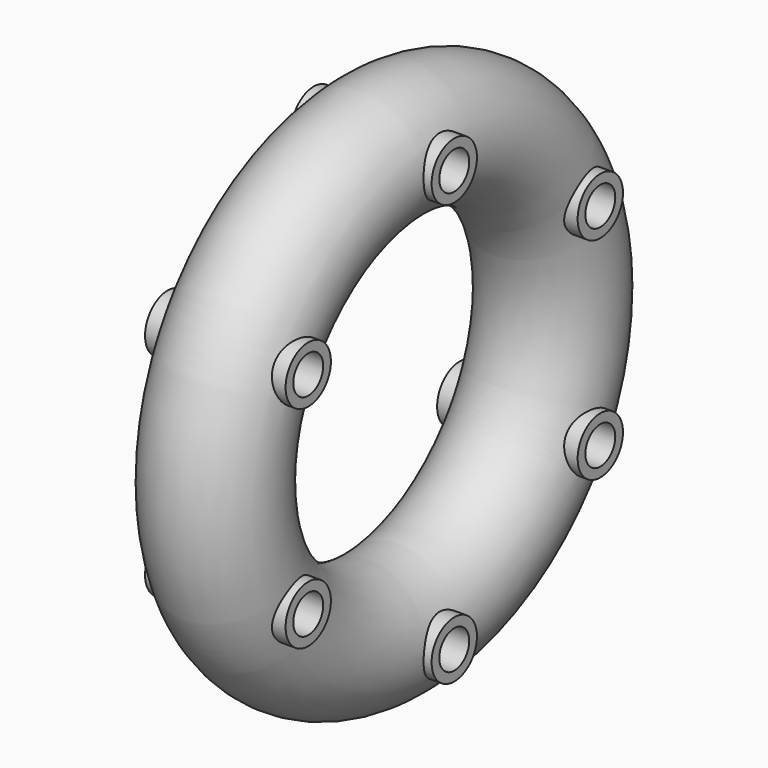
from build123d import *
from build123d import SkipClean  # not in build123d's __all__

# Parameters (mm, degrees)
F0_R          = 27.5
F2_R          = 12.5
F3_DEPTH      = 27.5010001
F3_DEPTH_BACK = 27.501
F4_R          = 12.5
F4_R_2        = 8.25
F5_DEPTH      = 31
F5_DEPTH_BACK = 31


with BuildPart() as f1:
    # F0 (on Front) → F1 (revolve)
    with BuildSketch(Plane.XZ):
        with Locations((0, 93)):
            Circle(F0_R)
    revolve(axis=Axis((3.4763067961, 0, 0), (1, 0, 0)))

    # F2 (on Right) → F3 (cut, two sides)
    with BuildSketch(Plane.YZ) as f3_sk:
        with Locations((0, 93)):
            Circle(F2_R)
        with Locations((-80.540362552, 46.5)):
            Circle(F2_R)
        with Locations((-80.540362552, -46.5)):
            Circle(F2_R)
        with Locations((0, -93)):
            Circle(F2_R)
        with Locations((80.540362552, -46.5)):
            Circle(F2_R)
        with Locations((80.540362552, 46.5)):
            Circle(F2_R)
    with SkipClean():  # cleaning this boolean's faces spoils the solid; the shape is the same uncleaned
        extrude(amount=-F3_DEPTH, mode=Mode.SUBTRACT)
        extrude(f3_sk.sketch, amount=F3_DEPTH_BACK, mode=Mode.SUBTRACT)


with BuildPart() as f5:
    # F4 (on Right) → F5 (new body, two sides)
    with BuildSketch(Plane.YZ) as f5_sk:
        with Locations((0, 93)):
            Circle(F4_R)
        with Locations((0, 93)):
            Circle(F4_R_2, mode=Mode.SUBTRACT)
    extrude(amount=F5_DEPTH)
    extrude(f5_sk.sketch, amount=-F5_DEPTH_BACK)


with BuildPart() as f5b:
    # F4 (on Right) → F5, piece 2 (new body, two sides)
    with BuildSketch(Plane.YZ) as f5_2_sk:
        with Locations((-80.540362552, 46.5)):
            Circle(F4_R)
        with Locations((-80.540362552, 46.5)):
            Circle(F4_R_2, mode=Mode.SUBTRACT)
    extrude(amount=F5_DEPTH)
    extrude(f5_2_sk.sketch, amount=-F5_DEPTH_BACK)


with BuildPart() as f5c:
    # F4 (on Right) → F5, piece 3 (new body, two sides)
    with BuildSketch(Plane.YZ) as f5_3_sk:
        with Locations((-80.540362552, -46.5)):
            Circle(F4_R)
        with Locations((-80.540362552, -46.5)):
            Circle(F4_R_2, mode=Mode.SUBTRACT)
    extrude(amount=F5_DEPTH)
    extrude(f5_3_sk.sketch, amount=-F5_DEPTH_BACK)


with BuildPart() as f5d:
    # F4 (on Right) → F5, piece 4 (new body, two sides)
    with BuildSketch(Plane.YZ) as f5_4_sk:
        with Locations((0, -93)):
            Circle(F4_R)
        with Locations((0, -93)):
            Circle(F4_R_2, mode=Mode.SUBTRACT)
    extrude(amount=F5_DEPTH)
    extrude(f5_4_sk.sketch, amount=-F5_DEPTH_BACK)


with BuildPart() as f5e:
    # F4 (on Right) → F5, piece 5 (new body, two sides)
    with BuildSketch(Plane.YZ) as f5_5_sk:
        with Locations((80.540362552, -46.5)):
            Circle(F4_R)
        with Locations((80.540362552, -46.5)):
            Circle(F4_R_2, mode=Mode.SUBTRACT)
    extrude(amount=F5_DEPTH)
    extrude(f5_5_sk.sketch, amount=-F5_DEPTH_BACK)


with BuildPart() as f5f:
    # F4 (on Right) → F5, piece 6 (new body, two sides)
    with BuildSketch(Plane.YZ) as f5_6_sk:
        with Locations((80.540362552, 46.5)):
            Circle(F4_R)
        with Locations((80.540362552, 46.5)):
            Circle(F4_R_2, mode=Mode.SUBTRACT)
    extrude(amount=F5_DEPTH)
    extrude(f5_6_sk.sketch, amount=-F5_DEPTH_BACK)


solid = Compound([f1.part, f5.part, f5b.part, f5c.part, f5d.part, f5e.part, f5f.part])
